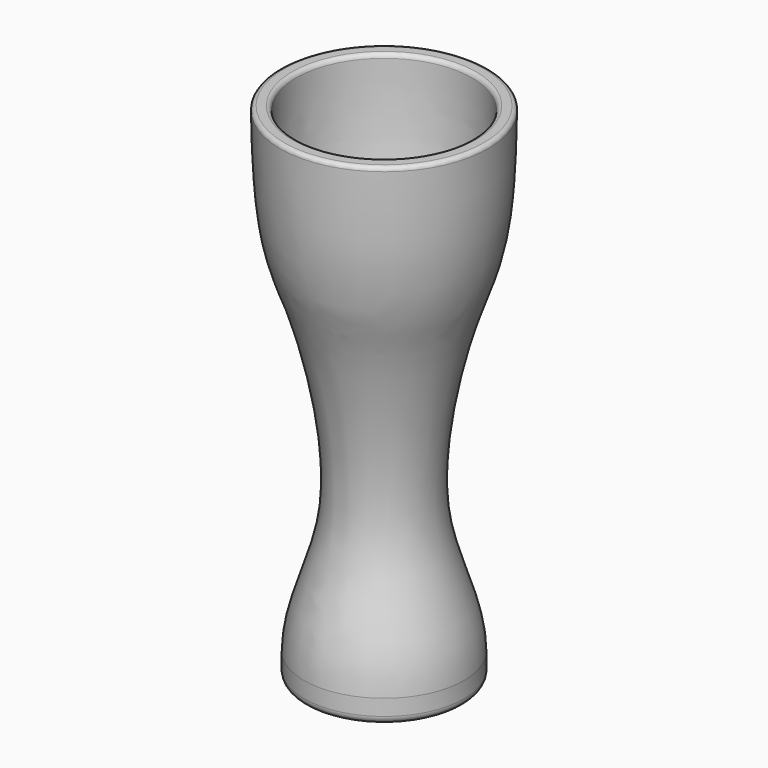
from build123d import *

# Parameters (mm, degrees)
F3_R         = 0.5
F4_R         = 1
F5_TEXT_SIZE = 11.1111111111
F6_DEPTH     = 2


# Not quite as in the source:
# - Text() gives the source's letters only with a copy of the font that has no kerning and outlines rounded to 1/6400 em; it was checked with that copy


with BuildPart() as f2:
    # F0 (on Right) → F2 (revolve)
    with BuildSketch(Plane.YZ):
        with BuildLine():
            Line((-11, 60), (-13, 60))
            add(Edge.make_bspline(
                [(-10, 0), (-9.8869893304, 5.5830442207), (-3.7310414184, 14.4294302617), (-9.6774690678, 41.3317198006), (-12.8705844246, 44.6239555716), (-13, 60)],
                knots=[0, 0, 0, 0, 0.2962312152, 0.6442565295, 1, 1, 1, 1], degree=3))
            Line((-10, 0), (-10, -3))
            Line((-10, -3), (0, -3))
            Line((0, -3), (0, 5))
            add(Edge.make_bspline(
                [(0, 5), (-1.4729600864, 5.0160666402), (-2.2867387227, 5.7816085239), (-3.0415283286, 8.3163303547), (-4.5489484228, 37.688455449), (-10.9931248572, 42.2494951353), (-11, 60)],
                knots=[0, 0, 0, 0, 0.1148090999, 0.2269722793, 0.5954691195, 1, 1, 1, 1], degree=3))
        make_face()
    revolve(axis=Axis((0, 0, 30.5088125169), (0, 0, 1)))

    # F3
    f3_edges = [f2.edges().sort_by_distance(p)[0] for p in [
        (0, 11, 60),
        (0, 13, 60),
    ]]
    fillet(f3_edges, radius=F3_R)

    # F4
    f4_edges = [f2.edges().sort_by_distance(p)[0] for p in [
        (0, 10, -3),
    ]]
    fillet(f4_edges, radius=F4_R)

    # F5 (on face) → F6 (cut)
    with BuildSketch(Plane(origin=(0, 0, -3), x_dir=(1, 0, 0), z_dir=(0, 0, -1))):
        with Locations((-5.8838611111, -4)):
            Text('Ju', F5_TEXT_SIZE, font='Arimo', text_align=(TextAlign.LEFT, TextAlign.BOTTOM))
    extrude(amount=-F6_DEPTH, mode=Mode.SUBTRACT)


solid = f2.part
